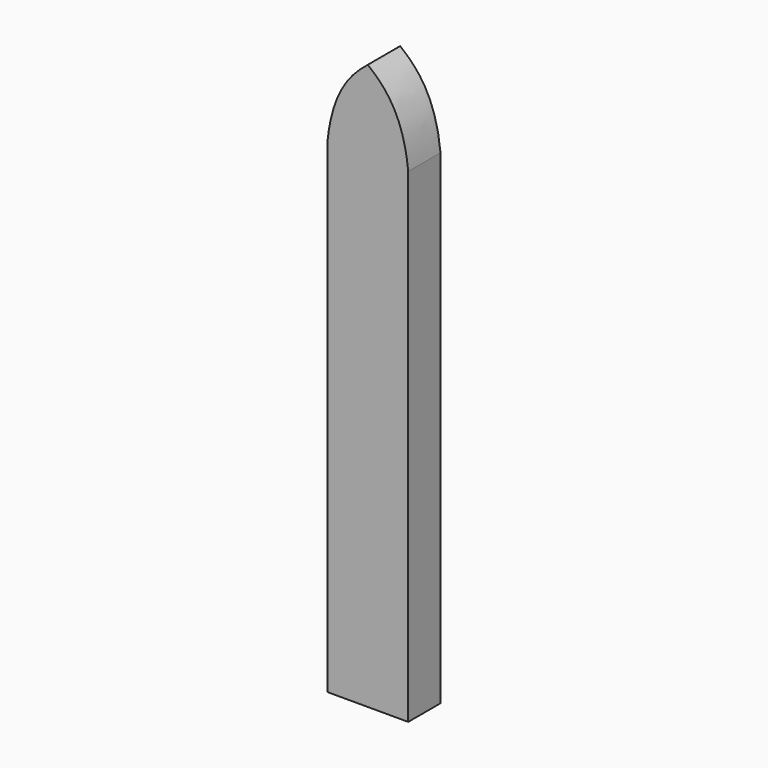
from build123d import *

# Parameters (mm, degrees)
F1_DEPTH      = 5
F2_DEPTH      = 25
F2_DEPTH_BACK = 74
F3_DEPTH      = 74
F3_DEPTH_BACK = 5.0010001


# Not quite as in the source:
# - an extrude ends at something that could not be found from the text; its depth is read off the source's solid


with BuildPart() as f1:
    # F0 (on Front) → F1 (new body)
    with BuildSketch(Plane.XZ):
        with BuildLine():
            add(Edge.make_bspline(
                [(5, 25), (4.3878769502, 31.0586858541), (1.9895534497, 33.4048718214), (0, 35)],
                knots=[0, 0, 0, 0, 11.1803398875, 11.1803398875, 11.1803398875, 11.1803398875], degree=3))
            add(Edge.make_bspline(
                [(-5, 25), (-4.3878769502, 31.0586858541), (-1.9895534497, 33.4048718214), (0, 35)],
                knots=[0, 0, 0, 0, 11.1803398875, 11.1803398875, 11.1803398875, 11.1803398875], degree=3))
            Line((-5, 25), (-5, -35))
            Line((-5, -35), (5, -35))
            Line((5, -35), (5, 25))
        make_face()
        with BuildLine():
            Line((5, 25), (5, 35))
            Line((5, 35), (0, 35))
            add(Edge.make_bspline(
                [(5, 25), (4.3878769502, 31.0586858541), (1.9895534497, 33.4048718214), (0, 35)],
                knots=[0, 0, 0, 0, 11.1803398875, 11.1803398875, 11.1803398875, 11.1803398875], degree=3))
        make_face()
        with BuildLine():
            add(Edge.make_bspline(
                [(-5, 25), (-4.3878769502, 31.0586858541), (-1.9895534497, 33.4048718214), (0, 35)],
                knots=[0, 0, 0, 0, 11.1803398875, 11.1803398875, 11.1803398875, 11.1803398875], degree=3))
            Line((0, 35), (-5, 35))
            Line((-5, 35), (-5, 25))
        make_face()
    extrude(amount=F1_DEPTH)

    # F0 (on Front) → F2 (cut, two sides)
    with BuildSketch(Plane.XZ) as f2_sk:
        with BuildLine():
            add(Edge.make_bspline(
                [(-5, 25), (-4.3878769502, 31.0586858541), (-1.9895534497, 33.4048718214), (0, 35)],
                knots=[0, 0, 0, 0, 11.1803398875, 11.1803398875, 11.1803398875, 11.1803398875], degree=3))
            Line((0, 35), (-5, 35))
            Line((-5, 35), (-5, 25))
        make_face()
    extrude(amount=F2_DEPTH, mode=Mode.SUBTRACT)
    extrude(f2_sk.sketch, amount=-F2_DEPTH_BACK, mode=Mode.SUBTRACT)

    # F0 (on Front) → F3 (cut, two sides)
    with BuildSketch(Plane.XZ) as f3_sk:
        with BuildLine():
            Line((5, 25), (5, 35))
            Line((5, 35), (0, 35))
            add(Edge.make_bspline(
                [(5, 25), (4.3878769502, 31.0586858541), (1.9895534497, 33.4048718214), (0, 35)],
                knots=[0, 0, 0, 0, 11.1803398875, 11.1803398875, 11.1803398875, 11.1803398875], degree=3))
        make_face()
    extrude(amount=-F3_DEPTH, mode=Mode.SUBTRACT)
    extrude(f3_sk.sketch, amount=F3_DEPTH_BACK, mode=Mode.SUBTRACT)


solid = f1.part
